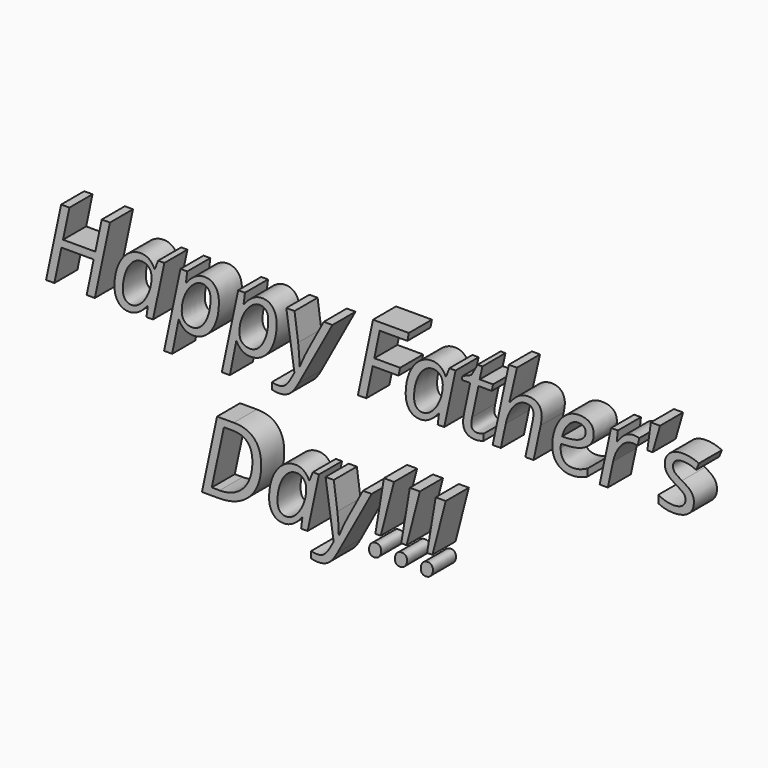
from build123d import *

# Parameters (mm, degrees)
F0_TEXT_SIZE = 8.8021282106
F1_DEPTH     = 2.54


# Not quite as in the source:
# - Text() gives the source's letters only with a copy of the font that has no kerning and outlines rounded to 1/6400 em; it was checked with that copy


with BuildPart() as f1:
    # F0 (on Front) → F1 (new body)
    with BuildSketch(Plane.XZ):
        with Locations((12.0128971499, 0)):
            Text("Happy Father's", F0_TEXT_SIZE, font='Open Sans', font_style=FontStyle.ITALIC, text_align=(TextAlign.LEFT, TextAlign.BOTTOM))
        with Locations((25.7359651632, -11.9708943664)):
            Text('Day!!!', F0_TEXT_SIZE, font='Open Sans', font_style=FontStyle.ITALIC, text_align=(TextAlign.LEFT, TextAlign.BOTTOM))
    extrude(amount=F1_DEPTH)


solid = f1.part
